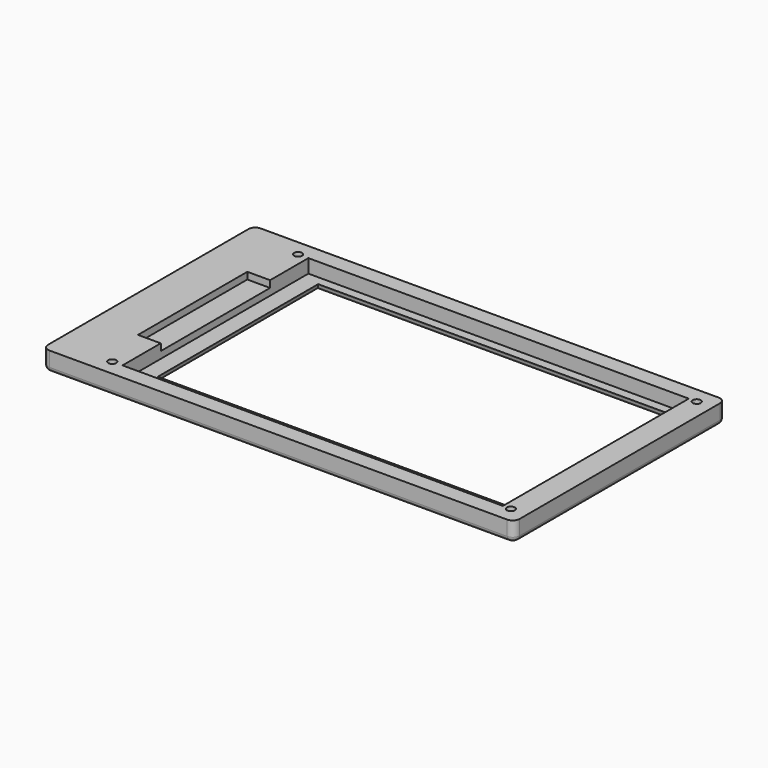
from build123d import *

# Parameters (mm, degrees)
F0_W      = 207
F0_H      = 116
F1_DEPTH  = 6
F2_W      = 167
F2_H      = 102
F3_DEPTH  = 6
F4_R      = 1.75
F5_DEPTH  = 25
F6_W      = 10
F6_H      = 60
F7_DEPTH  = 3
F8_W      = 207
F8_H      = 116
F8_R      = 1.75
F8_W_2    = 167
F8_H_2    = 102
F9_DEPTH  = 2.5
F10_W     = 155
F10_H     = 88
F11_DEPTH = 25
F13_R     = 3
F14_R     = 2


with BuildPart() as f1:
    # F0 (on Top) → F1 (new body)
    with BuildSketch(Plane.XY):
        with Locations((103.5, -58)):
            Rectangle(F0_W, F0_H)
    extrude(amount=F1_DEPTH)

    # F2 (on face) → F3 (cut)
    with BuildSketch(Plane.XY):
        with Locations((113, -58)):
            Rectangle(F2_W, F2_H)
    extrude(amount=F3_DEPTH, mode=Mode.SUBTRACT)

    # F4 (on face) → F5 (cut)
    with BuildSketch(Plane(origin=(0, 0, 0), x_dir=(1, 0, 0), z_dir=(0, 0, -1))):
        with Locations((200, 7)):
            Circle(F4_R)
        with Locations((200, 109)):
            Circle(F4_R)
        with Locations((25, 109)):
            Circle(F4_R)
        with Locations((25, 7)):
            Circle(F4_R)
    extrude(amount=-F5_DEPTH, mode=Mode.SUBTRACT)

    # F6 (on face) → F7 (cut)
    with BuildSketch(Plane.XY.offset(6)):
        with Locations((24.5, -58)):
            Rectangle(F6_W, F6_H)
    extrude(amount=-F7_DEPTH, mode=Mode.SUBTRACT)

    # F8 (on face) → F9 (join)
    with BuildSketch(Plane(origin=(0, 0, 0), x_dir=(1, 0, 0), z_dir=(0, 0, -1))):
        with Locations((103.5, 58)):
            Rectangle(F8_W, F8_H)
        with Locations((25, 7)):
            Circle(F8_R, mode=Mode.SUBTRACT)
        with Locations((200, 7)):
            Circle(F8_R, mode=Mode.SUBTRACT)
        with Locations((25, 109)):
            Circle(F8_R, mode=Mode.SUBTRACT)
        with Locations((113, 58)):
            Rectangle(F8_W_2, F8_H_2, mode=Mode.SUBTRACT)
        with Locations((200, 109)):
            Circle(F8_R, mode=Mode.SUBTRACT)
        with Locations((113, 58)):
            Rectangle(F8_W_2, F8_H_2)
    extrude(amount=F9_DEPTH)

    # F10 (on face) → F11 (cut)
    with BuildSketch(Plane(origin=(0, 0, -2.5), x_dir=(1, 0, 0), z_dir=(0, 0, -1))):
        with Locations((114.5, 55)):
            Rectangle(F10_W, F10_H)
    extrude(amount=-F11_DEPTH, mode=Mode.SUBTRACT)

    # F13
    f13_edges = [f1.edges().sort_by_distance(p)[0] for p in [
        (207, 0, 1.75),
        (0, 0, 1.75),
        (207, -116, 1.75),
        (0, -116, 1.75),
    ]]
    fillet(f13_edges, radius=F13_R)

    # F14
    f14_edges = [f1.edges().sort_by_distance(p)[0] for p in [
        (0, -58, -2.5),
        (114.5, -99, -2.5),
        (37, -55, -2.5),
        (192, -55, -2.5),
        (114.5, -11, -2.5),
        (103.5, 0, -2.5),
        (206.12132, -0.87868, -2.5),
        (0.87868, -0.87868, -2.5),
        (207, -58, -2.5),
        (0.87868, -115.12132, -2.5),
        (206.12132, -115.12132, -2.5),
        (103.5, -116, -2.5),
    ]]
    fillet(f14_edges, radius=F14_R)


solid = f1.part
